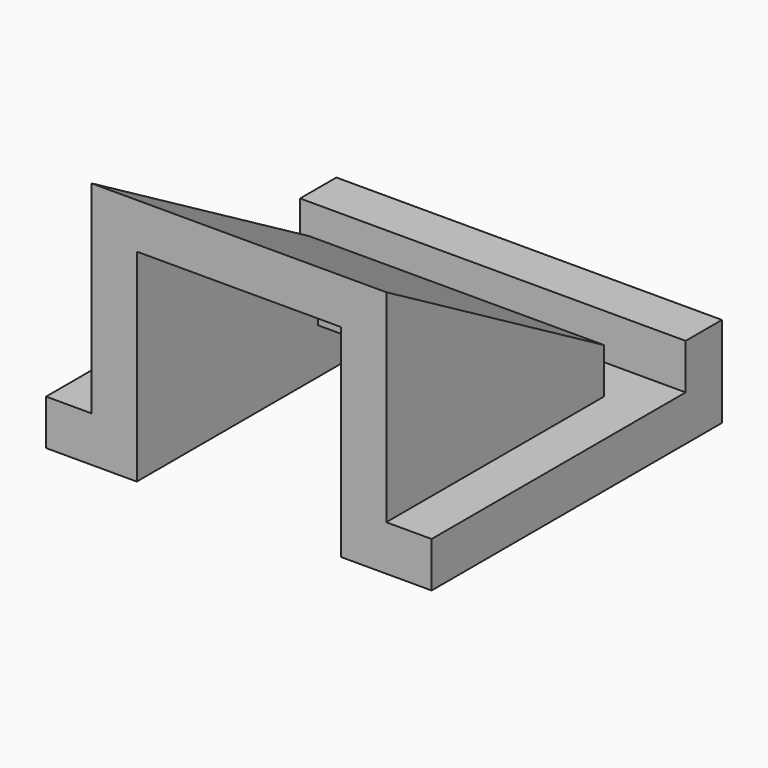
from build123d import *

# Parameters (mm, degrees)
F4_DEPTH  = 9
F6_DEPTH  = 2
F8_DEPTH  = 2
F9_W      = 9
F9_H      = 2
F10_DEPTH = 2
F11_W     = 17
F11_H     = 2
F12_DEPTH = 4


# Not quite as in the source:
# - a pattern or mirror of a feature is missing from the dataset's text; its kind, count and spacing are read off the source's solid


with BuildPart() as f4:
    # F3 (on plane+point) → F4 (new body, through all)
    with BuildSketch(Plane.YZ.offset(4.5)):
        Polygon((4.5, 0), (6.5, 0), (6.5, 4), (-5.5, 10.9282032303), (-5.5, 8.9282032303), (4.5, 3.1547005384), align=None)
    extrude(amount=-F4_DEPTH)

    # F5 (on face) → F6 (join)
    with BuildSketch(Plane.YZ.offset(4.5)):
        Polygon((6.5, 4), (-5.5, 10.9282032303), (-5.5, 0), (6.5, 0), align=None)
    f6 = extrude(amount=F6_DEPTH)

    # F6_copies: F6 across plane
    add(f6.mirror(Plane(origin=(0, 0, 0), x_dir=(0, 0, -1), z_dir=(-1, 0, 0))))

    # F7 (on Top) → F8 (join)
    with BuildSketch(Plane.XY):
        Polygon((4.5, 8.5), (4.5, 6.5), (6.5, 6.5), (6.5, -5.5), (8.5, -5.5), (8.5, 8.5), align=None)
    f8 = extrude(amount=F8_DEPTH)

    # F8_copies: F8 across plane
    add(f8.mirror(Plane(origin=(0, 0, 0), x_dir=(0, 0, -1), z_dir=(-1, 0, 0))))

    # F9 (on face) → F10 (cut, through all)
    with BuildSketch(Plane(origin=(0, 6.5, 0), x_dir=(-1, 0, 0), z_dir=(0, 1, 0))):
        with Locations((0, 1)):
            Rectangle(F9_W, F9_H)
    extrude(amount=-F10_DEPTH, mode=Mode.SUBTRACT)

    # F11 (on Top) → F12 (join)
    with BuildSketch(Plane.XY):
        with Locations((0, 9.5)):
            Rectangle(F11_W, F11_H)
    extrude(amount=F12_DEPTH)


solid = f4.part
